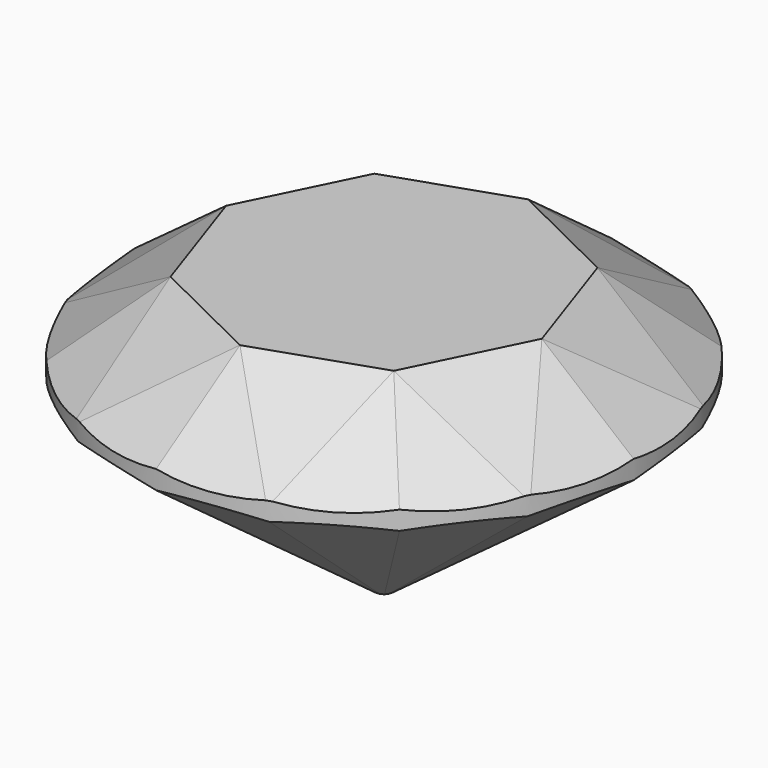
from build123d import *

# Parameters (mm, degrees)
F1_DEPTH               = 1.4278
DRAFT_F1_DRAFTED_ANGLE = 53
F2_DEPTH               = 0.0826
F3_DEPTH               = 0.561
F3_TAPER               = 53
F12_DEPTH              = 25
F12_COPIES_COUNT       = 8
F14_R                  = 1.96
F15_DEPTH              = 25


# Not quite as in the source:
# - an extrude with a draft is written as a straight extrude whose walls are then drafted
# - a pattern or mirror of a feature is missing from the dataset's text; its kind, count and spacing are read off the source's solid


with BuildPart() as f1:
    # F0 (on Top) → F1 (new body)
    with BuildSketch(Plane.XY):
        Polygon((1.8920140379, 0.6433351577), (1.5017993385, 1.3184066108), (0.8829493037, 1.7927626088), (0.1296782414, 1.9941867511), (-0.6433351577, 1.8920140379), (-1.3184066108, 1.5017993385), (-1.7927626088, 0.8829493037), (-1.9941867511, 0.1296782414), (-1.8920140379, -0.6433351577), (-1.5017993385, -1.3184066108), (-0.8829493037, -1.7927626088), (-0.1296782414, -1.9941867511), (0.6433351577, -1.8920140379), (1.3184066108, -1.5017993385), (1.7927626088, -0.8829493037), (1.9941867511, -0.1296782414), align=None)
    extrude(amount=-F1_DEPTH)

    # draft_F1_drafted
    draft_f1_drafted_walls = [f1.faces().sort_by_distance(p)[0] for p in [
        (0.9808708842, -1.6969066882, -0.9518666667),
        (1.5555846098, -1.1923743211, -0.9518666667),
        (1.89347468, -0.5063137725, -0.9518666667),
        (1.9431003945, 0.2568284581, -0.9518666667),
        (1.6969066882, 0.9808708842, -0.9518666667),
        (1.1923743211, 1.5555846098, -0.9518666667),
        (0.5063137725, 1.89347468, -0.9518666667),
        (-0.2568284581, 1.9431003945, -0.9518666667),
        (-0.9808708842, 1.6969066882, -0.9518666667),
        (-1.5555846098, 1.1923743211, -0.9518666667),
        (-1.89347468, 0.5063137725, -0.9518666667),
        (-1.9431003945, -0.2568284581, -0.9518666667),
        (-1.6969066882, -0.9808708842, -0.9518666667),
        (-1.1923743211, -1.5555846098, -0.9518666667),
        (-0.5063137725, -1.89347468, -0.9518666667),
        (0.2568284581, -1.9431003945, -0.9518666667),
    ]]
    draft(draft_f1_drafted_walls, neutral_plane=Plane(origin=(0, 0, 0), x_dir=(1, 0, 0), z_dir=(0, 0, -1)), angle=DRAFT_F1_DRAFTED_ANGLE)

    # F2 (add): a face of the model
    f2_faces = [f1.faces().sort_by_distance(p)[0] for p in [
        (0, 0, 0),
    ]]
    extrude(f2_faces, amount=F2_DEPTH)

    # F2_face (on face) → F3 (join)
    with BuildSketch(Plane.XY.offset(0.0826)):
        Polygon((0.6433351577, -1.8920140379), (1.3184066108, -1.5017993385), (1.7927626088, -0.8829493037), (1.9941867511, -0.1296782414), (1.8920140379, 0.6433351577), (1.5017993385, 1.3184066108), (0.8829493037, 1.7927626088), (0.1296782414, 1.9941867511), (-0.6433351577, 1.8920140379), (-1.3184066108, 1.5017993385), (-1.7927626088, 0.8829493037), (-1.9941867511, 0.1296782414), (-1.8920140379, -0.6433351577), (-1.5017993385, -1.3184066108), (-0.8829493037, -1.7927626088), (-0.1296782414, -1.9941867511), align=None)
    extrude(amount=F3_DEPTH, taper=F3_TAPER)

    # F11 (on 3pt) → F12 (cut)
    with BuildSketch(Plane(origin=(0.2831764432, 0.5749686159, 0.9749704782), x_dir=(0.9701009432, -0.1232866518, -0.2090563598), z_dir=(-0.2427017925, -0.4927878609, -0.8356171157))):
        Polygon((0.6182581975, -1.5022754625), (0.6681679486, -0.3773520245), (-0.2090032417, -0.738349919), align=None)
    f12 = extrude(amount=-F12_DEPTH, mode=Mode.SUBTRACT)

    # F12_copies: F12 ×8 about axis
    f12_copies_axis = Axis((0, 0, 0), (0, 0, 1))
    for i in range(1, F12_COPIES_COUNT):
        add(f12.rotate(f12_copies_axis, i * 360 / F12_COPIES_COUNT), mode=Mode.SUBTRACT)

    # F14 (on face) → F15 (intersect)
    with BuildSketch(Plane.XY.offset(0.6436)):
        Circle(F14_R)
    extrude(amount=-F15_DEPTH, mode=Mode.INTERSECT)


solid = f1.part
